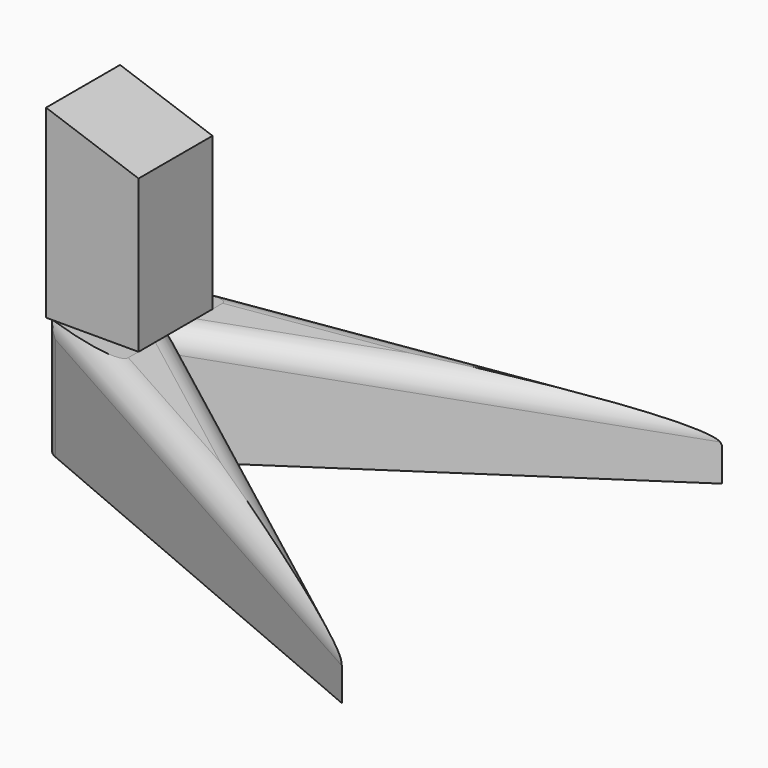
from build123d import *

# Parameters (mm, degrees)
F1_DEPTH      = 20
F2_DEPTH      = 25
F4_DEPTH      = 40
F6_DEPTH      = 61.3939463923
F8_DEPTH      = 84.6
F11_T1_DEPTH  = 41.5178477753
F11_T3_DEPTH  = 137.9615849437
F11_T5_DEPTH  = 137.9615849437
F11_T10_DEPTH = 139.2179253021
F11_T15_DEPTH = 139.2179253021
F11_T21_DEPTH = 139.2179253021
F11_T27_DEPTH = 139.2179253021


# Not quite as in the source:
# - a fillet or chamfer that OpenCascade refuses, or shapes differently, is made with other operations: its cross-section is extruded or revolved along the edge and cut away or added
# - a feature of the source that left no trace in its solid (it failed there, or was rolled back) is left out


with BuildPart() as f1:
    # F0 (on Top) → F1 (new body)
    with BuildSketch(Plane.XY):
        Polygon((87.0753377676, -51.3929463923), (10, 0), (10, -10), (-10, -10), align=None)
        Polygon((10, 0), (10, 10), (-10, 10), (-10, -10), (10, -10), align=None)
        Polygon((-10, 10), (10, 10), (10, 0), (87.0753377676, 51.3929463923), align=None)
    extrude(amount=F1_DEPTH)

    # F0 (on Top) → F2 (join)
    with BuildSketch(Plane.XY):
        Polygon((10, 0), (10, 10), (-10, 10), (-10, -10), (10, -10), align=None)
        Polygon((-10, 10), (10, 10), (10, 0), (87.0753377676, 51.3929463923), align=None)
        Polygon((87.0753377676, -51.3929463923), (10, 0), (10, -10), (-10, -10), align=None)
    extrude(amount=F2_DEPTH)

    # F7 (on Front) → F8 (cut, symmetric)
    with BuildSketch(Plane.XZ):
        Polygon((87.0753377676, 25), (10, 25), (87.0753377676, 12.5), align=None)
    extrude(amount=F8_DEPTH, both=True, mode=Mode.SUBTRACT)

    # F11: fillet of radius 5 on 6 edges, made by hand

    # F11_s2 → F11_t1 (cut)
    with BuildSketch(Plane.XY.offset(-8.2589238876)):
        with BuildLine():
            ThreePointArc((-6.9611566724, -11.2957634951), (-9.1716773222, -9.452715684), (-10, -6.6964304449))
            Line((-10, -6.6964304449), (-10, -10))
            Line((-10, -10), (-6.9611566724, -11.2957634951))
        make_face()
        with BuildLine():
            ThreePointArc((-10, 6.6964304449), (-9.1716773222, 9.452715684), (-6.9611566724, 11.2957634951))
            Line((-6.9611566724, 11.2957634951), (-10, 10))
            Line((-10, 10), (-10, 6.6964304449))
        make_face()
    extrude(amount=F11_T1_DEPTH, mode=Mode.SUBTRACT)

    # F11_s4 → F11_t3 (cut)
    with BuildSketch(Plane(origin=(100.6464893313, -42.9156862419, -16.3227454213), x_dir=(-0.3922313345, -0.91986661, 0), z_dir=(-0.909798278, 0.3879381954, 0.1475501607))):
        with BuildLine():
            ThreePointArc((13.1209794451, 21.83145176), (11.5437136037, 25.4762961846), (7.8070230934, 26.821585166))
            Line((7.8070230934, 26.821585166), (13.1209794451, 27.1559149751))
            Line((13.1209794451, 27.1559149751), (13.1209794451, 21.83145176))
        make_face()
    extrude(amount=F11_T3_DEPTH, mode=Mode.SUBTRACT)

    # F11_s6 → F11_t5 (cut)
    with BuildSketch(Plane(origin=(-24.87072308, -10.604882052, 4.0335086099), x_dir=(-0.3922313345, 0.91986661, 0), z_dir=(0.909798278, 0.3879381954, -0.1475501607))):
        with BuildLine():
            ThreePointArc((13.1209794451, 21.83145176), (11.5437136037, 25.4762961846), (7.8070230934, 26.821585166))
            Line((7.8070230934, 26.821585166), (13.1209794451, 27.1559149751))
            Line((13.1209794451, 27.1559149751), (13.1209794451, 21.83145176))
        make_face()
    extrude(amount=F11_T5_DEPTH, mode=Mode.SUBTRACT)


with BuildPart() as f4:
    # F3 (on face) → F4 (new body)
    with BuildSketch(Plane.XY.offset(25)):
        Polygon((10, 10), (-10, 10), (-10, -10), (10, -10), (10, 0), align=None)
    extrude(amount=F4_DEPTH)

    # F5 (on face) → F6 (cut, through all)
    with BuildSketch(Plane.XZ.offset(10)):
        Polygon((10, 65), (-10, 65), (10, 58.0052025616), align=None)
    extrude(amount=-F6_DEPTH, mode=Mode.SUBTRACT)


with BuildPart() as f11_tool8:
    # F11_s9 → F11_t10 (new body)
    with BuildSketch(Plane(origin=(-24.2435670935, 16.1653309616, 3.931797089), x_dir=(0.5547703521, 0.8320035195, 0), z_dir=(0.8245312391, -0.5497879218, -0.133721639))):
        with BuildLine():
            ThreePointArc((5.5477035213, 21.3140260519), (4.2368967072, 24.6889117739), (0.9917620666, 26.2942682155))
            Line((0.9917620666, 26.2942682155), (5.5477035213, 25.8880420385))
            Line((5.5477035213, 25.8880420385), (5.5477035213, 21.3140260519))
        make_face()
    extrude(amount=F11_T10_DEPTH)

    split(bisect_by=Plane(origin=(3.077701436, -4.6157088547, 0), x_dir=(0, 0, 1), z_dir=(0.5547703521, -0.8320035195, 0)), keep=Keep.TOP)


with BuildPart() as f1_1:
    add(f1.part)

    # F11_t7: cut F11_tool8
    add(f11_tool8.part, mode=Mode.SUBTRACT)


with BuildPart() as f11_tool13:
    # F11_s14 → F11_t15 (new body)
    with BuildSketch(Plane(origin=(90.5459613675, 60.3750028658, -14.6846520544), x_dir=(0.5547703521, -0.8320035195, 0), z_dir=(-0.8245312391, -0.5497879218, 0.133721639))):
        with BuildLine():
            ThreePointArc((5.5477035213, 21.3140260519), (4.2368967072, 24.6889117739), (0.9917620666, 26.2942682155))
            Line((0.9917620666, 26.2942682155), (5.5477035213, 25.8880420385))
            Line((5.5477035213, 25.8880420385), (5.5477035213, 21.3140260519))
        make_face()
    extrude(amount=F11_T15_DEPTH)

    split(bisect_by=Plane(origin=(3.077701436, 4.6157088547, 0), x_dir=(0, 0, 1), z_dir=(0.5547703521, 0.8320035195, 0)), keep=Keep.TOP)


with BuildPart() as f1_2:
    add(f1_1.part)

    # F11_t12: cut F11_tool13
    add(f11_tool13.part, mode=Mode.SUBTRACT)


with BuildPart() as f11_tool19:
    # F11_s20 → F11_t21 (new body)
    with BuildSketch(Plane(origin=(-24.2435670935, 16.1653309616, 3.931797089), x_dir=(0.5547703521, 0.8320035195, 0), z_dir=(0.8245312391, -0.5497879218, -0.133721639))):
        with BuildLine():
            ThreePointArc((5.5477035213, 21.3140260519), (4.2368967072, 24.6889117739), (0.9917620666, 26.2942682155))
            Line((0.9917620666, 26.2942682155), (5.5477035213, 25.8880420385))
            Line((5.5477035213, 25.8880420385), (5.5477035213, 21.3140260519))
        make_face()
    extrude(amount=F11_T21_DEPTH)

    split(bisect_by=Plane(origin=(3.077701436, -4.6157088547, 0), x_dir=(0, 0, 1), z_dir=(-0.5547703521, 0.8320035195, 0)), keep=Keep.TOP)

    split(bisect_by=Plane.XY.offset(25), keep=Keep.BOTTOM)

    split(bisect_by=Plane(origin=(-5.1464592774, 12.0695508825, 0), x_dir=(0, 0, 1), z_dir=(0.3922313345, -0.91986661, 0)), keep=Keep.TOP)


with BuildPart() as f11_tool25:
    # F11_s26 → F11_t27 (new body)
    with BuildSketch(Plane(origin=(90.5459613675, 60.3750028658, -14.6846520544), x_dir=(0.5547703521, -0.8320035195, 0), z_dir=(-0.8245312391, -0.5497879218, 0.133721639))):
        with BuildLine():
            ThreePointArc((5.5477035213, 21.3140260519), (4.2368967072, 24.6889117739), (0.9917620666, 26.2942682155))
            Line((0.9917620666, 26.2942682155), (5.5477035213, 25.8880420385))
            Line((5.5477035213, 25.8880420385), (5.5477035213, 21.3140260519))
        make_face()
    extrude(amount=F11_T27_DEPTH)

    split(bisect_by=Plane(origin=(3.077701436, 4.6157088547, 0), x_dir=(0, 0, 1), z_dir=(-0.5547703521, -0.8320035195, 0)), keep=Keep.TOP)

    split(bisect_by=Plane(origin=(-5.1464592774, -12.0695508825, 0), x_dir=(0, 0, 1), z_dir=(0.3922313345, 0.91986661, 0)), keep=Keep.TOP)

    split(bisect_by=Plane.XY.offset(25), keep=Keep.BOTTOM)


with BuildPart() as f11_tool19_1:
    add(f11_tool19.part)

    # F11_t31: intersect F11_tool25
    add(f11_tool25.part, mode=Mode.INTERSECT)


with BuildPart() as f1_3:
    add(f1_2.part)

    # F11_t17: cut F11_tool19
    add(f11_tool19_1.part, mode=Mode.SUBTRACT)


solid = Compound([f4.part, f1_3.part])
